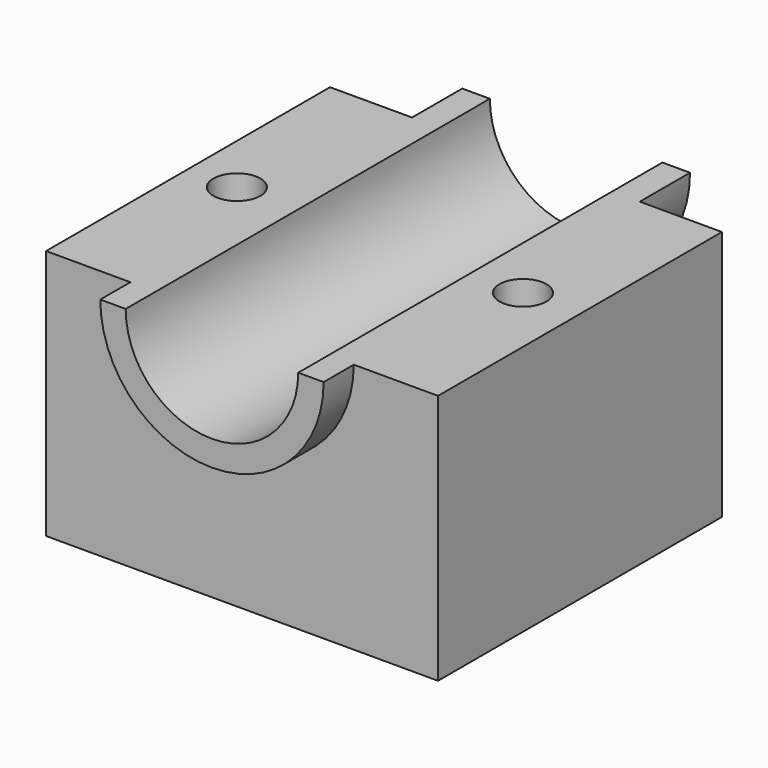
from build123d import *

# Parameters (mm, degrees)
F0_W      = 79.3684571981
F0_H      = 71.8531981111
F1_DEPTH  = 25.4
F2_DEPTH  = 25.4
F4_DEPTH  = 101.6
F5_R      = 4.7587178315
F6_DEPTH  = 127
F7_DEPTH  = 508
F9_DEPTH  = 7.62
F11_DEPTH = 25.4
F12_DEPTH = 12.7


with BuildPart() as f1:
    # F0 (on Top) → F1 (new body)
    with BuildSketch(Plane.XY):
        Rectangle(F0_W, F0_H)
    extrude(amount=F1_DEPTH)

    # F2 (add): a face of the model
    f2_faces = [f1.faces().sort_by_distance(p)[0] for p in [
        (0, 0, 25.4),
    ]]
    extrude(f2_faces, amount=F2_DEPTH)

    # F3 (on face) → F4 (cut)
    with BuildSketch(Plane.XZ.offset(35.9265990555)):
        with BuildLine():
            ThreePointArc((-17.4702548625, 50.8), (0, 33.3297451375), (17.4702548625, 50.8))
            Line((17.4702548625, 50.8), (-17.4702548625, 50.8))
        make_face()
    extrude(amount=-F4_DEPTH, mode=Mode.SUBTRACT)

    # F5 (on face) → F6 (join)
    with BuildSketch(Plane.XY.offset(50.8)):
        with Locations((-29.7860819846, 0)):
            Circle(F5_R)
        with Locations((28.1363911927, 0)):
            Circle(F5_R)
    extrude(amount=F6_DEPTH)

    # F7 (cut): faces of the model
    f7_faces = [f1.faces().sort_by_distance(p)[0] for p in [
        (28.1363911927, 0, 177.8),
        (-29.7860819846, 0, 177.8),
    ]]
    extrude(f7_faces, amount=-F7_DEPTH, mode=Mode.SUBTRACT)

    # F8 (on face) → F9 (join)
    with BuildSketch(Plane.XZ.offset(35.9265990555)):
        with BuildLine():
            Line((-17.4702548625, 50.8), (-22.6149617575, 50.8))
            ThreePointArc((-22.6149617575, 50.8), (0, 28.1850382425), (22.6149617575, 50.8))
            Line((22.6149617575, 50.8), (17.4702548625, 50.8))
            ThreePointArc((17.4702548625, 50.8), (0, 33.3297451375), (-17.4702548625, 50.8))
        make_face()
    extrude(amount=F9_DEPTH)

    # F10 (on face) → F11 (join)
    with BuildSketch(Plane(origin=(0, 35.9265990555, 0), x_dir=(-1, 0, 0), z_dir=(0, 1, 0))):
        with BuildLine():
            Line((-17.4702548625, 50.8), (-23.0630593563, 50.8))
            ThreePointArc((-23.0630593563, 50.8), (0, 27.7369406437), (23.0630593563, 50.8))
            Line((23.0630593563, 50.8), (17.4702548625, 50.8))
            ThreePointArc((17.4702548625, 50.8), (0, 33.3297451375), (-17.4702548625, 50.8))
        make_face()
    extrude(amount=F11_DEPTH)

    # F12 (cut): a face of the model
    f12_faces = [f1.faces().sort_by_distance(p)[0] for p in [
        (20.2666571094, 61.3265990555, 50.2842943151),
    ]]
    extrude(f12_faces, amount=-F12_DEPTH, mode=Mode.SUBTRACT)


solid = f1.part
